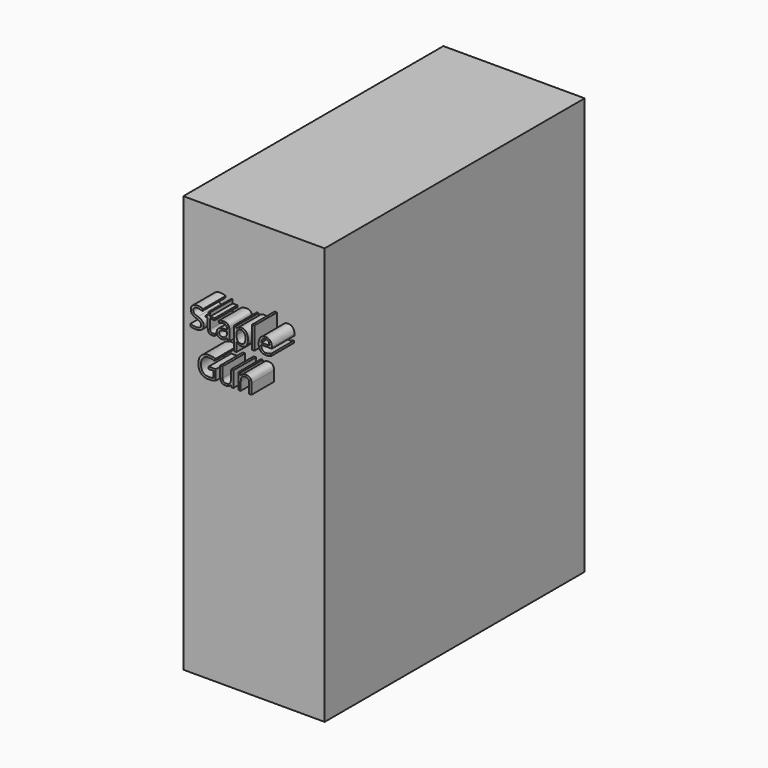
from build123d import *

# Parameters (mm, degrees)
F0_W         = 127
F0_H         = 374.65
F1_DEPTH     = 292.1
F2_TEXT_SIZE = 26.2999514642
F3_DEPTH     = 25.4


# Not quite as in the source:
# - Text() gives the source's letters only with a copy of the font that has no kerning and outlines rounded to 1/6400 em; it was checked with that copy


with BuildPart() as f1:
    # F0 (on Front) → F1 (new body)
    with BuildSketch(Plane.XZ):
        Rectangle(F0_W, F0_H)
    extrude(amount=F1_DEPTH)

    # F2 (on face) → F3 (join)
    with BuildSketch(Plane.XZ.offset(292.1)):
        with Locations((-38.1, 102.7708463672)):
            Text('Staple', F2_TEXT_SIZE, font='Open Sans', text_align=(TextAlign.LEFT, TextAlign.BOTTOM))
        with Locations((-31.2661219867, 67.0029123759)):
            Text('Gun', F2_TEXT_SIZE, font='Open Sans', text_align=(TextAlign.LEFT, TextAlign.BOTTOM))
    extrude(amount=F3_DEPTH)


solid = f1.part
